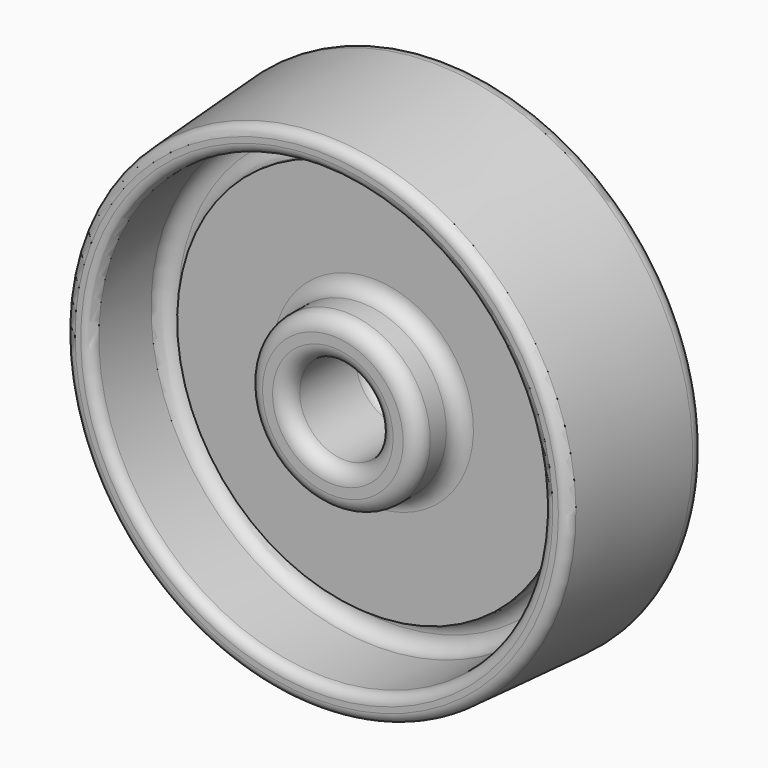
from build123d import *

# Parameters (mm, degrees)
F3_D = 5
F4_R = 1.49999
F5_R = 1


# Not quite as in the source:
# - a fillet or chamfer is up to 0.001 mm smaller than in the source, because OpenCascade refuses the exact size


with BuildPart() as f1:
    # F0 (on Right) → F1 (revolve)
    with BuildSketch(Plane.YZ):
        Polygon((-4, 0), (0, 0), (0, 26), (-16, 25), (-16, 22.5), (-7, 22.5), (-7, 19.5), (-9, 19.5), (-9, 8.5), (-14, 8.5), (-14, 4.5), (-4, 4.5), align=None)
    revolve(axis=Axis((0, -2, 0), (0, -1, 0)))

    # F3 (through all)
    with Locations(Plane(origin=(0, 0, 0), x_dir=(-1, 0, 0), z_dir=(0, 1, 0))):
        with Locations((0, 0)):
            Hole(F3_D / 2)

    # F4 (radius 1.5 in the source; OpenCascade refuses exactly that, so slightly less here)
    f4_edges = [f1.edges().sort_by_distance(p)[0] for p in [
        (0, -14, -8.5),
        (0, -14, -4.5),
        (0, -7, -22.5),
        (0, -7, -19.5),
        (0, 0, -26),
        (0, -4, -4.5),
        (0, -9, -8.5),
        (2.5, 0, 0),
    ]]
    fillet(f4_edges, radius=F4_R)

    # F5
    f5_edges = [f1.edges().sort_by_distance(p)[0] for p in [
        (0, -16, -25),
        (0, -16, -22.5),
    ]]
    fillet(f5_edges, radius=F5_R)


solid = f1.part
